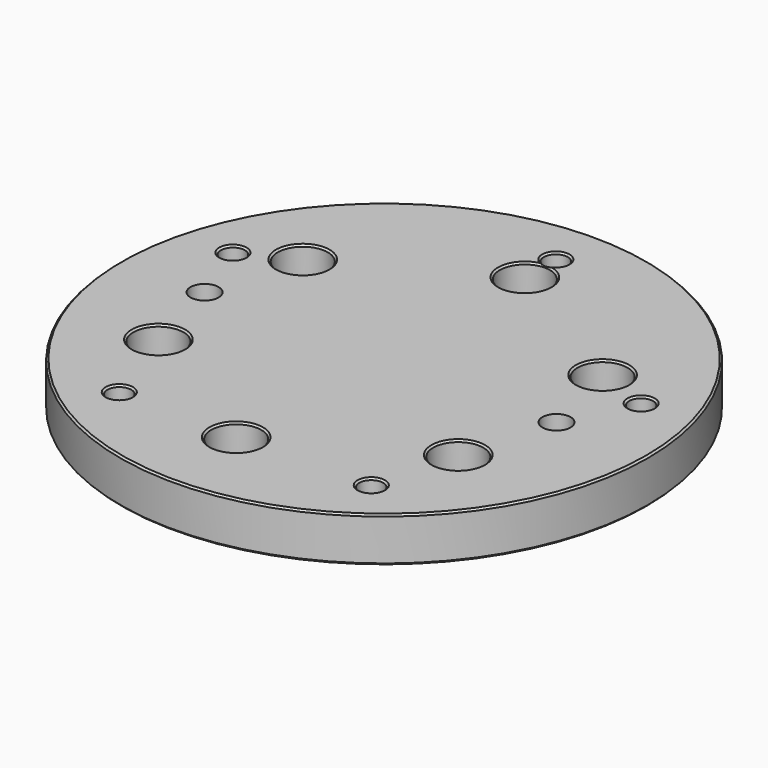
from build123d import *

# Parameters (mm, degrees)
F0_R           = 75
F1_DEPTH       = 12.7
F2_D           = 6.8
F4_D           = 9
F4_CBORE_D     = 14.25
F4_CBORE_DEPTH = 8
F6_D           = 8


# Not quite as in the source:
# - a fillet or chamfer that OpenCascade refuses, or shapes differently, is made with other operations: its cross-section is extruded or revolved along the edge and cut away or added


with BuildPart() as f1:
    # F0 (on Top) → F1 (new body)
    with BuildSketch(Plane.XY):
        Circle(F0_R)
    extrude(amount=F1_DEPTH)

    # F2 (through all)
    with Locations(Plane(origin=(0, 0, 0), x_dir=(1, 0, 0), z_dir=(0, 0, -1))):
        with Locations((-58, -18.8), (0, -61), (58, -18.8), (35.8, 49.3), (-35.8, 49.3)):
            Hole(F2_D / 2)

    # F4 (through all)
    with Locations(Plane.XY.offset(12.7)):
        with Locations((0, 50), (-43.8068557852, 25.8756999398), (42.7956845933, 24.1243000602), (-44.8180269771, -24.1243000602), (-2.0223423839, -50), (41.7845134013, -25.8756999398)):
            CounterBoreHole(F4_D / 2, F4_CBORE_D / 2, F4_CBORE_DEPTH)

    # F5: chamfer of 0.5 on 24 edges, made by hand

    # F5_s1 → F5_t2 (revolve, cut)
    with BuildSketch(Plane.XZ):
        Polygon((75, 12.2), (74.5, 12.7), (75, 12.7), align=None)
    revolve(axis=Axis((0, 0, 12.7), (0, 0, 1)), mode=Mode.SUBTRACT)

    # F5_s3 → F5_t4 (revolve, cut)
    with BuildSketch(Plane.XZ.offset(49.3)):
        Polygon((-31.9, 12.7), (-32.4, 12.2), (-32.4, 12.7), align=None)
    revolve(axis=Axis((-35.8, -49.3, 12.7), (0, 0, -1)), mode=Mode.SUBTRACT)

    # F5_s5 → F5_t6 (revolve, cut)
    with BuildSketch(Plane.XZ.offset(50)):
        Polygon((5.6026576161, 12.7), (5.1026576161, 12.2), (5.1026576161, 12.7), align=None)
    revolve(axis=Axis((-2.0223423839, -50, 12.7), (0, 0, 1)), mode=Mode.SUBTRACT)

    # F5_s7 → F5_t8 (revolve, cut)
    with BuildSketch(Plane.XZ.offset(24.1243000602)):
        Polygon((-37.1930269771, 12.7), (-37.6930269771, 12.2), (-37.6930269771, 12.7), align=None)
    revolve(axis=Axis((-44.8180269771, -24.1243000602, 12.7), (0, 0, 1)), mode=Mode.SUBTRACT)

    # F5_s9 → F5_t10 (revolve, cut)
    with BuildSketch(Plane.XZ.offset(49.3)):
        Polygon((39.7, 12.7), (39.2, 12.2), (39.2, 12.7), align=None)
    revolve(axis=Axis((35.8, -49.3, 12.7), (0, 0, -1)), mode=Mode.SUBTRACT)

    # F5_s11 → F5_t12 (revolve, cut)
    with BuildSketch(Plane.XZ.offset(25.8756999398)):
        Polygon((49.4095134013, 12.7), (48.9095134013, 12.2), (48.9095134013, 12.7), align=None)
    revolve(axis=Axis((41.7845134013, -25.8756999398, 12.7), (0, 0, 1)), mode=Mode.SUBTRACT)

    # F5_s13 → F5_t14 (revolve, cut)
    with BuildSketch(Plane.XZ.offset(-18.8)):
        Polygon((-54.1, 12.7), (-54.6, 12.2), (-54.6, 12.7), align=None)
    revolve(axis=Axis((-58, 18.8, 12.7), (0, 0, -1)), mode=Mode.SUBTRACT)

    # F5_s15 → F5_t16 (revolve, cut)
    with BuildSketch(Plane.XZ.offset(-25.8756999398)):
        Polygon((-36.1818557852, 12.7), (-36.6818557852, 12.2), (-36.6818557852, 12.7), align=None)
    revolve(axis=Axis((-43.8068557852, 25.8756999398, 12.7), (0, 0, 1)), mode=Mode.SUBTRACT)

    # F5_s17 → F5_t18 (revolve, cut)
    with BuildSketch(Plane.XZ.offset(-18.8)):
        Polygon((61.9, 12.7), (61.4, 12.2), (61.4, 12.7), align=None)
    revolve(axis=Axis((58, 18.8, 12.7), (0, 0, -1)), mode=Mode.SUBTRACT)

    # F5_s19 → F5_t20 (revolve, cut)
    with BuildSketch(Plane.XZ.offset(-24.1243000602)):
        Polygon((50.4206845933, 12.7), (49.9206845933, 12.2), (49.9206845933, 12.7), align=None)
    revolve(axis=Axis((42.7956845933, 24.1243000602, 12.7), (0, 0, 1)), mode=Mode.SUBTRACT)

    # F5_s21 → F5_t22 (revolve, cut)
    with BuildSketch(Plane.XZ.offset(-50)):
        Polygon((7.625, 12.7), (7.125, 12.2), (7.125, 12.7), align=None)
    revolve(axis=Axis((0, 50, 12.7), (0, 0, 1)), mode=Mode.SUBTRACT)

    # F5_s23 → F5_t24 (revolve, cut)
    with BuildSketch(Plane.XZ.offset(-61)):
        Polygon((3.9, 12.7), (3.4, 12.2), (3.4, 12.7), align=None)
    revolve(axis=Axis((0, 61, 12.7), (0, 0, -1)), mode=Mode.SUBTRACT)

    # F5_s25 → F5_t26 (revolve, cut)
    with BuildSketch(Plane.XZ):
        Polygon((75, 0.5), (74.5, 0), (75, 0), align=None)
    revolve(axis=Axis((0, 0, 0), (0, 0, 1)), mode=Mode.SUBTRACT)

    # F5_s27 → F5_t28 (revolve, cut)
    with BuildSketch(Plane.XZ.offset(49.3)):
        Polygon((-31.9, 0), (-32.4, 0.5), (-32.4, 0), align=None)
    revolve(axis=Axis((-35.8, -49.3, 0), (0, 0, -1)), mode=Mode.SUBTRACT)

    # F5_s29 → F5_t30 (revolve, cut)
    with BuildSketch(Plane.XZ.offset(50)):
        Polygon((2.9776576161, 0), (2.4776576161, 0.5), (2.4776576161, 0), align=None)
    revolve(axis=Axis((-2.0223423839, -50, 0), (0, 0, 1)), mode=Mode.SUBTRACT)

    # F5_s31 → F5_t32 (revolve, cut)
    with BuildSketch(Plane.XZ.offset(24.1243000602)):
        Polygon((-39.8180269771, 0), (-40.3180269771, 0.5), (-40.3180269771, 0), align=None)
    revolve(axis=Axis((-44.8180269771, -24.1243000602, 0), (0, 0, 1)), mode=Mode.SUBTRACT)

    # F5_s33 → F5_t34 (revolve, cut)
    with BuildSketch(Plane.XZ.offset(49.3)):
        Polygon((39.7, 0), (39.2, 0.5), (39.2, 0), align=None)
    revolve(axis=Axis((35.8, -49.3, 0), (0, 0, -1)), mode=Mode.SUBTRACT)

    # F5_s35 → F5_t36 (revolve, cut)
    with BuildSketch(Plane.XZ.offset(25.8756999398)):
        Polygon((46.7845134013, 0), (46.2845134013, 0.5), (46.2845134013, 0), align=None)
    revolve(axis=Axis((41.7845134013, -25.8756999398, 0), (0, 0, 1)), mode=Mode.SUBTRACT)

    # F5_s37 → F5_t38 (revolve, cut)
    with BuildSketch(Plane.XZ.offset(-18.8)):
        Polygon((-54.1, 0), (-54.6, 0.5), (-54.6, 0), align=None)
    revolve(axis=Axis((-58, 18.8, 0), (0, 0, -1)), mode=Mode.SUBTRACT)

    # F5_s39 → F5_t40 (revolve, cut)
    with BuildSketch(Plane.XZ.offset(-25.8756999398)):
        Polygon((-38.8068557852, 0), (-39.3068557852, 0.5), (-39.3068557852, 0), align=None)
    revolve(axis=Axis((-43.8068557852, 25.8756999398, 0), (0, 0, 1)), mode=Mode.SUBTRACT)

    # F5_s41 → F5_t42 (revolve, cut)
    with BuildSketch(Plane.XZ.offset(-18.8)):
        Polygon((61.9, 0), (61.4, 0.5), (61.4, 0), align=None)
    revolve(axis=Axis((58, 18.8, 0), (0, 0, -1)), mode=Mode.SUBTRACT)

    # F5_s43 → F5_t44 (revolve, cut)
    with BuildSketch(Plane.XZ.offset(-24.1243000602)):
        Polygon((47.7956845933, 0), (47.2956845933, 0.5), (47.2956845933, 0), align=None)
    revolve(axis=Axis((42.7956845933, 24.1243000602, 0), (0, 0, 1)), mode=Mode.SUBTRACT)

    # F5_s45 → F5_t46 (revolve, cut)
    with BuildSketch(Plane.XZ.offset(-50)):
        Polygon((5, 0), (4.5, 0.5), (4.5, 0), align=None)
    revolve(axis=Axis((0, 50, 0), (0, 0, 1)), mode=Mode.SUBTRACT)

    # F5_s47 → F5_t48 (revolve, cut)
    with BuildSketch(Plane.XZ.offset(-61)):
        Polygon((3.9, 0), (3.4, 0.5), (3.4, 0), align=None)
    revolve(axis=Axis((0, 61, 0), (0, 0, -1)), mode=Mode.SUBTRACT)

    # F6 (through all)
    with Locations(Plane.XY.offset(12.7)):
        with Locations((-51.0111711919, 0), (48.9888288081, 0)):
            Hole(F6_D / 2)


solid = f1.part
